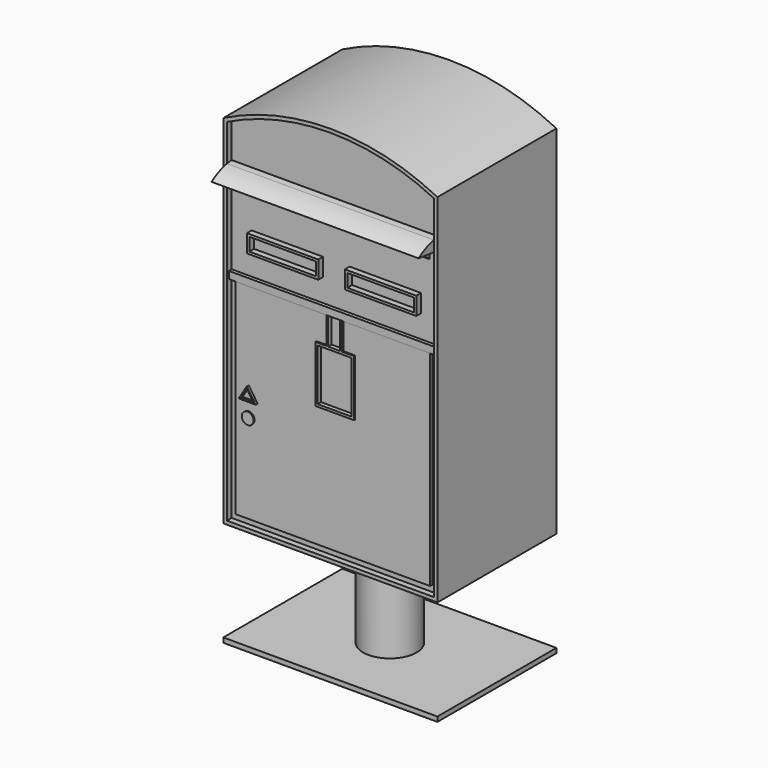
from build123d import *

# Parameters (mm, degrees)
F1_DEPTH  = 600
F2_T      = -5
F4_DEPTH  = 25
F5_W      = 300
F5_H      = 75
F5_W_2    = 280
F5_H_2    = 55
F6_DEPTH  = 25
F7_W      = 870
F7_H      = 30
F8_DEPTH  = 15
F9_W      = 142.9338163137
F9_H      = 217.2664716095
F10_DEPTH = 18
F12_DEPTH = 12
F13_R     = 24.8551421214
F14_DEPTH = 5
F16_DEPTH = 10
F18_DEPTH = 870
F20_DEPTH = 20
F22_DEPTH = 18
F25_DEPTH = 5
F27_DEPTH = 5
F28_W     = 391.7387041664
F28_H     = 69.7681009769
F28_W_2   = 377.2408955904
F29_DEPTH = 25
F30_R     = 112.5
F31_DEPTH = 422
F32_W     = 900
F32_H     = 625
F32_R     = 112.5
F33_DEPTH = 20


with BuildPart() as f1:
    # F0 (on Front) → F1 (new body)
    with BuildSketch(Plane.XZ):
        with BuildLine():
            Line((-450, -750), (450, -750))
            Line((450, -750), (450, 750))
            ThreePointArc((450, 750), (0, 856.9714450254), (-450, 750))
            Line((-450, 750), (-450, -750))
        make_face()
    extrude(amount=F1_DEPTH)

    # F2
    f2_openings = [f1.faces().sort_by_distance(p)[0] for p in [
        (0, 0, 36.375009),
    ]]
    offset(amount=F2_T, openings=f2_openings)

    # F3 (on face) → F4 (join)
    with BuildSketch(Plane.XZ.offset(600)):
        with BuildLine():
            Line((450, -750), (450, 750))
            ThreePointArc((450, 750), (0, 856.9714450254), (-450, 750))
            Line((-450, 750), (-450, -750))
            Line((-450, -750), (450, -750))
        make_face()
        with BuildLine():
            Line((435, 740.7134888368), (435, -735))
            Line((435, -735), (-435, -735))
            Line((-435, -735), (-435, 740.7134888368))
            ThreePointArc((-435, 740.7134888368), (0, 841.9714450254), (435, 740.7134888368))
        make_face(mode=Mode.SUBTRACT)
    extrude(amount=F4_DEPTH)

    # F5 (on face) → F6 (join)
    with BuildSketch(Plane.XZ.offset(600)):
        with Locations((-200.8810852704, 318.7295198674)):
            Rectangle(F5_W, F5_H)
        with Locations((-200.8810852704, 318.7295198674)):
            Rectangle(F5_W_2, F5_H_2, mode=Mode.SUBTRACT)
        with Locations((211.2015885351, 318.7295198674)):
            Rectangle(F5_W, F5_H)
        with Locations((211.2015885351, 318.7295198674)):
            Rectangle(F5_W_2, F5_H_2, mode=Mode.SUBTRACT)
    extrude(amount=F6_DEPTH)

    # F7 (on face) → F8 (join)
    with BuildSketch(Plane.XZ.offset(600)):
        with Locations((0, 170.2089005709)):
            Rectangle(F7_W, F7_H)
    extrude(amount=F8_DEPTH)

    # F9 (on face) → F10 (join)
    with BuildSketch(Plane.XZ.offset(600)):
        Polygon((-14.5836101339, 155.2089005709), (-22.9078065604, 155.2089005709), (-22.9078065604, 42.8976975381), (-69.0468810499, 42.8976975381), (-69.0468810499, -194.3687740713), (93.8869352639, -194.3687740713), (93.8869352639, 42.8976975381), (44.0564386487, 42.8976975381), (44.0564386487, 155.2089005709), (34.6765947954, 155.2089005709), (34.6765947954, 42.8976975381), (-14.5836101339, 42.8976975381), align=None)
        with Locations((12.420027107, -75.7355382666)):
            Rectangle(F9_W, F9_H, mode=Mode.SUBTRACT)
    extrude(amount=F10_DEPTH)

    # F11 (on face) → F12 (join)
    with BuildSketch(Plane.XZ.offset(600)):
        Polygon((-22.9078065604, 155.2089005709), (-408.6377620697, 155.2089005709), (-408.6377620697, -707.8300118446), (408.7606370449, -707.8300118446), (408.7606370449, 155.2089005709), (44.0564386487, 155.2089005709), (44.0564386487, 42.8976975381), (93.8869352639, 42.8976975381), (93.8869352639, -194.3687740713), (-69.0468810499, -194.3687740713), (-69.0468810499, 42.8976975381), (-22.9078065604, 42.8976975381), align=None)
    extrude(amount=F12_DEPTH)

    # F13 (on face) → F14 (join)
    with BuildSketch(Plane.XZ.offset(612)):
        with Locations((-354.0675938129, -333.6301445961)):
            Circle(F13_R)
    extrude(amount=F14_DEPTH)

    # F15 (on face) → F16 (join)
    with BuildSketch(Plane.XZ.offset(612)):
        Polygon((-387.899610247, -268.6794745922), (-316.3461361468, -268.6794745922), (-353.5931451269, -212.8089411077), align=None)
        Polygon((-378.9620697498, -263.6794745922), (-353.4200489521, -222.0824658871), (-325.6887197495, -263.6794745922), align=None, mode=Mode.SUBTRACT)
    extrude(amount=F16_DEPTH)

    # F17 (on face) → F18 (join, through all)
    with BuildSketch(Plane.YZ.offset(-435)):
        with BuildLine():
            Line((-625, 577.9839080805), (-625, 586.1312416531))
            ThreePointArc((-625, 586.1312416531), (-667.0829642918, 573.1979535583), (-705.2572369576, 551.2669086456))
            Line((-705.2572369576, 551.2669086456), (-693.4141296704, 549.7889105873))
            ThreePointArc((-693.4141296704, 549.7889105873), (-660.5960632562, 567.2567631744), (-625, 577.9839080805))
        make_face()
        with BuildLine():
            Line((-600, 581.2005341429), (-600, 589.2150402069))
            ThreePointArc((-600, 589.2150402069), (-612.5491949312, 588.0719585758), (-625, 586.1312416531))
            Line((-625, 586.1312416531), (-625, 577.9839080805))
            ThreePointArc((-625, 577.9839080805), (-612.5535193278, 580.008179687), (-600, 581.2005341429))
        make_face()
    extrude(amount=F18_DEPTH)

    # F19 (on face) → F20 (join)
    with BuildSketch(Plane.YZ.offset(435)):
        with BuildLine():
            ThreePointArc((-625, 577.9839080805), (-660.5960632562, 567.2567631744), (-693.4141296704, 549.7889105873))
            Line((-693.4141296704, 549.7889105873), (-600, 538.1309986115))
            Line((-600, 538.1309986115), (-600, 589.2150402069))
            ThreePointArc((-600, 589.2150402069), (-612.5491949312, 588.0719585758), (-625, 586.1312416531))
            Line((-625, 586.1312416531), (-625, 577.9839080805))
        make_face()
        with BuildLine():
            ThreePointArc((-625, 586.1312416531), (-667.0829642918, 573.1979535583), (-705.2572369576, 551.2669086456))
            Line((-705.2572369576, 551.2669086456), (-693.4141296704, 549.7889105873))
            ThreePointArc((-693.4141296704, 549.7889105873), (-660.5960632562, 567.2567631744), (-625, 577.9839080805))
            Line((-625, 577.9839080805), (-625, 586.1312416531))
        make_face()
    extrude(amount=-F20_DEPTH)

    # F21 (on face) → F22 (join)
    with BuildSketch(Plane(origin=(-435, 0, 0), x_dir=(0, -1, 0), z_dir=(-1, 0, 0))):
        with BuildLine():
            ThreePointArc((625, 577.9839080805), (660.5960632562, 567.2567631744), (693.4141296704, 549.7889105873))
            Line((693.4141296704, 549.7889105873), (705.2572369576, 551.2669086456))
            ThreePointArc((705.2572369576, 551.2669086456), (667.0829642918, 573.1979535583), (625, 586.1312416531))
            Line((625, 586.1312416531), (625, 577.9839080805))
        make_face()
        with BuildLine():
            Line((600, 589.2150402069), (600, 581.2005341429))
            Line((600, 581.2005341429), (600, 538.1309986115))
            Line((600, 538.1309986115), (693.4141296704, 549.7889105873))
            ThreePointArc((693.4141296704, 549.7889105873), (660.5960632562, 567.2567631744), (625, 577.9839080805))
            Line((625, 577.9839080805), (625, 586.1312416531))
            ThreePointArc((625, 586.1312416531), (612.5491949312, 588.0719585758), (600, 589.2150402069))
        make_face()
    extrude(amount=-F22_DEPTH)

    # F24 (on offset) → F25 (join)
    with BuildSketch(Plane.YZ):
        with BuildLine():
            Line((-600, 538.1309986115), (-600, 581.2005341429))
            ThreePointArc((-600, 581.2005341429), (-648.7839740291, 571.6711832668), (-693.4141296704, 549.7889105873))
            Line((-693.4141296704, 549.7889105873), (-600, 538.1309986115))
        make_face()
    extrude(amount=F25_DEPTH)

    # F26 (on face) → F27 (join)
    with BuildSketch(Plane(origin=(0, 0, 0), x_dir=(-1, 0, 0), z_dir=(0, 1, 0))):
        with BuildLine():
            ThreePointArc((445, 746.9152634769), (0, 851.9714450254), (-445, 746.9152634769))
            Line((-445, 746.9152634769), (-445, -745))
            Line((-445, -745), (445, -745))
            Line((445, -745), (445, 746.9152634769))
        make_face()
    extrude(amount=-F27_DEPTH)

    # F28 (on face) → F29 (cut)
    with BuildSketch(Plane.XZ.offset(600)):
        with Locations((-207.7159030628, 527.7101248503)):
            Rectangle(F28_W, F28_H)
        with Locations((208.6599989108, 527.7101248503)):
            Rectangle(F28_W_2, F28_H)
    extrude(amount=-F29_DEPTH, mode=Mode.SUBTRACT)

    # F30 (on face) → F31 (join)
    with BuildSketch(Plane(origin=(0, 0, -750), x_dir=(1, 0, 0), z_dir=(0, 0, -1))):
        with Locations((0, 312.5)):
            Circle(F30_R)
    extrude(amount=F31_DEPTH)

    # F32 (on face) → F33 (join)
    with BuildSketch(Plane(origin=(0, 0, -1172), x_dir=(1, 0, 0), z_dir=(0, 0, -1))):
        with Locations((0, 312.5)):
            Rectangle(F32_W, F32_H)
        with Locations((0, 312.5)):
            Circle(F32_R, mode=Mode.SUBTRACT)
        with Locations((0, 312.5)):
            Circle(F32_R)
    extrude(amount=F33_DEPTH)


solid = f1.part
